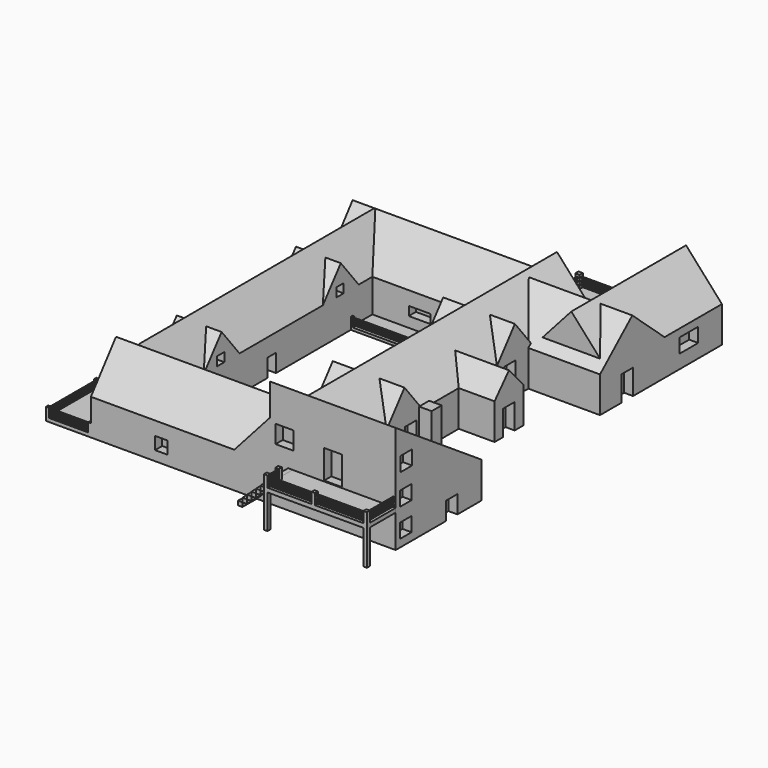
from build123d import *

# Parameters (mm, degrees)
F0_W       = 101.6
F0_H       = 50.8
F1_DEPTH   = 508
F2_W       = 152.4
F2_H       = 50.8
F3_DEPTH   = 127
F4_DEPTH   = 127
F5_DEPTH   = 50.8
F6_W       = 50.8
F6_H       = 50.8
F7_DEPTH   = 50.8
F8_DEPTH   = 25.4
F9_W       = 114.3
F9_H       = 50.8
F10_DEPTH  = 101.6
F11_DEPTH  = 50.8
F12_W      = 101.6
F12_H      = 50.8
F13_DEPTH  = 101.6
F14_DEPTH  = 101.6
F15_W      = 88.9
F15_H      = 50.8
F16_DEPTH  = 203.2
F17_DEPTH  = 50.8
F18_DEPTH  = 50.8
F19_W      = 63.5
F19_H      = 50.8
F20_DEPTH  = 355.6
F21_DEPTH  = 17.78
F22_DEPTH  = 43.18
F24_DEPTH  = 101.6
F26_DEPTH  = 63.5
F27_W      = 101.6
F27_H      = 7.62
F28_DEPTH  = 101.6
F29_W      = 6.096
F29_H      = 5.588
F30_DEPTH  = 17.78
F31_W      = 1.524
F31_H      = 1.397
F32_DEPTH  = 63.5
F33_W      = 1.524
F33_H      = 1.397
F34_DEPTH  = 127
F35_W      = 5.08
F35_H      = 3.81
F36_DEPTH  = 30.48
F37_W      = 6.35
F37_H      = 5.842
F38_DEPTH  = 25.4
F37_W_2    = 146.05
F39_DEPTH  = 50.8
F40_W      = 5.08
F40_H      = 5.08
F41_DEPTH  = 15.24
F42_W      = 1.778
F42_H      = 1.778
F43_DEPTH  = 139.7
F44_W      = 1.778
F44_H      = 1.778
F45_DEPTH  = 50.8
F46_W      = 1.778
F46_H      = 1.778
F47_DEPTH  = 17.78
F48_W      = 330.2
F48_H      = 3.81
F49_DEPTH  = 38.1
F50_W      = 101.6
F50_H      = 3.81
F51_DEPTH  = 38.1
F52_W      = 101.6
F52_H      = 3.81
F53_DEPTH  = 38.1
F54_W      = 15.24
F54_H      = 2.54
F55_DEPTH  = 2.54
F56_W      = 3.048
F56_H      = 3.048
F57_DEPTH  = 12.7
F58_W      = 1.27
F58_H      = 1.27
F62_DEPTH  = 101.6
F59_W      = 1.27
F59_H      = 1.27
F63_DEPTH  = 109.22
F60_W      = 1.27
F60_H      = 1.27
F64_DEPTH  = 127
F61_W      = 1.27
F61_H      = 1.27
F65_DEPTH  = 101.6
F66_W      = 17.78
F66_H      = 17.78
F67_DEPTH  = 114.3
F70_DEPTH  = 63.5
F69_W      = 20.32
F69_H      = 38.1
F69_W_2    = 17.78
F69_H_2    = 17.78
F69_W_3    = 17.272
F69_H_3    = 35.56
F78_DEPTH  = 12.7
F71_W      = 20.32
F71_H      = 35.56
F71_W_2    = 12.7
F71_H_2    = 12.7
F79_DEPTH  = 12.7
F72_W      = 40.64
F72_H      = 15.24
F80_DEPTH  = 12.7
F73_W      = 33.02
F73_H      = 20.32
F81_DEPTH  = 12.7
F74_W      = 20.32
F74_H      = 35.56
F74_W_2    = 33.02
F74_H_2    = 20.32
F82_DEPTH  = 12.7
F75_W      = 20.32
F75_H      = 20.32
F83_DEPTH  = 12.7
F76_W      = 20.32
F76_H      = 35.56
F84_DEPTH  = 12.7
F77_W      = 20.32
F77_H      = 20.32
F77_H_2    = 25.4
F85_DEPTH  = 12.7
F68_W      = 25.4
F68_H      = 25.4
F68_H_2    = 40.64
F86_DEPTH  = 12.7
F87_W      = 20.32
F87_H      = 25.4
F87_W_2    = 15.24
F87_H_2    = 15.24
F91_DEPTH  = 12.7
F88_W      = 30.48
F88_H      = 12.7
F92_DEPTH  = 12.7
F89_W      = 12.7
F89_H      = 12.7
F89_W_2    = 15.24
F89_H_2    = 25.4
F93_DEPTH  = 12.7
F90_W      = 30.48
F90_H      = 12.7
F94_DEPTH  = 12.7
F95_W      = 3.81
F95_H      = 3.81
F96_DEPTH  = 12.7
F97_W      = 1.524
F97_H      = 1.524
F100_DEPTH = 58.42
F99_W      = 1.524
F99_H      = 1.524
F101_DEPTH = 81.28
F98_W      = 1.524
F98_H      = 1.524
F102_DEPTH = 58.42
F103_W     = 3.81
F103_H     = 3.81
F104_DEPTH = 12.7
F105_W     = 1.524
F105_H     = 1.524
F108_DEPTH = 58.42
F106_W     = 1.524
F106_H     = 1.524
F109_DEPTH = 83.82
F107_W     = 1.524
F107_H     = 1.524
F110_DEPTH = 58.42
F111_W     = 5.08
F111_H     = 5.08
F112_DEPTH = 48.26
F68_W_2    = 17.78
F68_H_3    = 17.78
F113_DEPTH = 12.7


# Not quite as in the source:
# - a feature names something its author has since deleted; it is built from what else it names


with BuildPart() as f1:
    # F0 (on Front) → F1 (new body)
    with BuildSketch(Plane.XZ):
        Polygon((0, 56.7961266285), (-50.8, 0), (50.8, 0), align=None)
        with Locations((0, -25.4)):
            Rectangle(F0_W, F0_H)
    extrude(amount=F1_DEPTH)

    # F2 (on face) → F3 (join)
    with BuildSketch(Plane.YZ.offset(50.8)):
        with Locations((-431.8, -25.4)):
            Rectangle(F2_W, F2_H)
    extrude(amount=F3_DEPTH)

    # F2 (on face) → F4 (join)
    with BuildSketch(Plane.YZ.offset(50.8)):
        Polygon((-508, 0), (-355.6, 0), (-508, 101.6), align=None)
    extrude(amount=F4_DEPTH)

    # F5 (add): a face of the model
    f5_faces = [f1.faces().sort_by_distance(p)[0] for p in [
        (50.8, -457.2, 33.8666666667),
    ]]
    extrude(f5_faces, amount=F5_DEPTH)

    # F6 (on face) → F7 (join)
    with BuildSketch(Plane.YZ.offset(50.8)):
        with Locations((-212.1169992447, -25.4)):
            Rectangle(F6_W, F6_H)
        Polygon((-212.1169992447, 28.3980633142), (-237.5169992447, 0), (-186.7169992447, 0), align=None)
    extrude(amount=F7_DEPTH)

    # F8 (add): a face of the model
    f8_faces = [f1.faces().sort_by_distance(p)[0] for p in [
        (50.8, -212.1169992447, 9.4660211047),
    ]]
    extrude(f8_faces, amount=F8_DEPTH)

    # F9 (on face) → F10 (join)
    with BuildSketch(Plane.YZ.offset(50.8)):
        Polygon((-57.15, 50.4015624758), (-114.3, 0), (0, 0), align=None)
        with Locations((-57.15, -25.4)):
            Rectangle(F9_W, F9_H)
    extrude(amount=F10_DEPTH)

    # F11 (add): a face of the model
    f11_faces = [f1.faces().sort_by_distance(p)[0] for p in [
        (50.8, -57.15, 16.8005208253),
    ]]
    extrude(f11_faces, amount=F11_DEPTH)

    # F12 (on face) → F13 (join)
    with BuildSketch(Plane(origin=(0, 0, 0), x_dir=(-1, 0, 0), z_dir=(0, 1, 0))):
        with Locations((-101.6, -25.4)):
            Rectangle(F12_W, F12_H)
        Polygon((-152.4, 0), (-50.8, 0), (-101.6, 56.7961266285), align=None)
    extrude(amount=F13_DEPTH)

    # F14 (add): a face of the model
    f14_faces = [f1.faces().sort_by_distance(p)[0] for p in [
        (101.6, 0, 18.9320422095),
    ]]
    extrude(f14_faces, amount=F14_DEPTH)

    # F15 (on face) → F16 (join)
    with BuildSketch(Plane(origin=(-50.8, 0, 0), x_dir=(0, -1, 0), z_dir=(-1, 0, 0))):
        with Locations((44.45, -25.4)):
            Rectangle(F15_W, F15_H)
        Polygon((44.45, 56.8137306995), (0, 0), (88.9, 0), align=None)
        with Locations((463.55, -25.4)):
            Rectangle(F15_W, F15_H)
        Polygon((463.55, 56.8137306995), (419.1, 0), (508, 0), align=None)
    extrude(amount=F16_DEPTH)

    # F17 (add): a face of the model
    f17_faces = [f1.faces().sort_by_distance(p)[0] for p in [
        (-50.8, -44.45, 18.9379102332),
    ]]
    extrude(f17_faces, amount=F17_DEPTH)

    # F18 (add): a face of the model
    f18_faces = [f1.faces().sort_by_distance(p)[0] for p in [
        (-50.8, -463.55, 18.9379102332),
    ]]
    extrude(f18_faces, amount=F18_DEPTH)

    # F19 (on face) → F20 (join)
    with BuildSketch(Plane.XZ.offset(88.9)):
        with Locations((-222.25, -25.4)):
            Rectangle(F19_W, F19_H)
        Polygon((-254, 0), (-190.5, 0), (-222.25, 57.6171441153), align=None)
    extrude(amount=F20_DEPTH)

    # F21 (add): a face of the model
    f21_faces = [f1.faces().sort_by_distance(p)[0] for p in [
        (-222.25, -444.5, 40.8490406859),
    ]]
    extrude(f21_faces, amount=F21_DEPTH)

    # F22 (add): a face of the model
    f22_faces = [f1.faces().sort_by_distance(p)[0] for p in [
        (-222.25, -88.9, 19.2057147051),
    ]]
    extrude(f22_faces, amount=F22_DEPTH)

    # F23 (on face) → F24 (join)
    with BuildSketch(Plane(origin=(-50.8, 0, 0), x_dir=(0, -1, 0), z_dir=(-1, 0, 0))):
        Polygon((138.0952139497, 39.6557372898), (106.3452139497, 0), (169.8452139497, 0), align=None)
        Polygon((333.6137141702, 39.6557372898), (301.8637141702, 0), (365.3637141702, 0), align=None)
    extrude(amount=-F24_DEPTH)

    # F25 (on face) → F26 (join)
    with BuildSketch(Plane(origin=(-254, 0, 0), x_dir=(0, -1, 0), z_dir=(-1, 0, 0))):
        Polygon((144.8305835128, 39.6557372898), (113.0805835128, 0), (176.5805835128, 0), align=None)
        Polygon((355.9101884365, 39.6557372898), (324.1601884365, 0), (387.6601884365, 0), align=None)
    extrude(amount=-F26_DEPTH)

    # F27 (on face) → F28 (join)
    with BuildSketch(Plane(origin=(50.8, 0, 0), x_dir=(0, -1, 0), z_dir=(-1, 0, 0))):
        with Locations((-50.8, -46.99)):
            Rectangle(F27_W, F27_H)
    extrude(amount=F28_DEPTH)

    # F29 (on face) → F30 (join)
    with BuildSketch(Plane.XY.offset(-43.18)):
        with Locations((-47.752, 33.3146086487)):
            Rectangle(F29_W, F29_H)
        with Locations((-47.752, 98.806)):
            Rectangle(F29_W, F29_H)
        with Locations((6.6813429161, 98.806)):
            Rectangle(F29_W, F29_H)
    extrude(amount=F30_DEPTH)

    # F31 (on face) → F32 (join)
    with BuildSketch(Plane(origin=(0, 36.1086086487, 0), x_dir=(-1, 0, 0), z_dir=(0, 1, 0))):
        with Locations((47.498, -38.7985)):
            Rectangle(F31_W, F31_H)
        with Locations((47.498, -34.0995)):
            Rectangle(F31_W, F31_H)
        with Locations((47.498, -29.4005)):
            Rectangle(F31_W, F31_H)
    extrude(amount=F32_DEPTH)

    # F33 (on face) → F34 (join)
    with BuildSketch(Plane.YZ.offset(-44.704)):
        with Locations((98.806, -29.4005)):
            Rectangle(F33_W, F33_H)
        with Locations((98.806, -34.0995)):
            Rectangle(F33_W, F33_H)
        with Locations((98.806, -38.7985)):
            Rectangle(F33_W, F33_H)
    extrude(amount=F34_DEPTH)

    # F35 (on face) → F36 (join)
    with BuildSketch(Plane(origin=(0, 0, 0), x_dir=(-1, 0, 0), z_dir=(0, 1, 0))):
        with Locations((53.34, -48.895)):
            Rectangle(F35_W, F35_H)
    extrude(amount=F36_DEPTH)

    # F48 (on face) → F49 (join)
    with BuildSketch(Plane(origin=(-50.8, 0, 0), x_dir=(0, -1, 0), z_dir=(-1, 0, 0))):
        with Locations((254, -48.895)):
            Rectangle(F48_W, F48_H)
    extrude(amount=F49_DEPTH)

    # F50 (on face) → F51 (join)
    with BuildSketch(Plane.XZ.offset(88.9)):
        with Locations((-139.7, -48.895)):
            Rectangle(F50_W, F50_H)
    extrude(amount=F51_DEPTH)

    # F52 (on face) → F53 (join)
    with BuildSketch(Plane(origin=(0, -419.1, 0), x_dir=(-1, 0, 0), z_dir=(0, 1, 0))):
        with Locations((139.7, -48.895)):
            Rectangle(F52_W, F52_H)
    extrude(amount=F53_DEPTH)

    # F54 (on face) → F55 (join)
    with BuildSketch(Plane(origin=(-88.9, 0, 0), x_dir=(0, -1, 0), z_dir=(-1, 0, 0))):
        with Locations((246.4711151075, -49.53)):
            Rectangle(F54_W, F54_H)
    extrude(amount=F55_DEPTH)

    # F56 (on face) → F57 (join)
    with BuildSketch(Plane.XY.offset(-46.99)):
        with Locations((-188.976, -125.476)):
            Rectangle(F56_W, F56_H)
        with Locations((-87.376, -125.476)):
            Rectangle(F56_W, F56_H)
        with Locations((-87.376, -237.3516275177)):
            Rectangle(F56_W, F56_H)
        with Locations((-87.376, -255.524)):
            Rectangle(F56_W, F56_H)
        with Locations((-87.376, -382.524)):
            Rectangle(F56_W, F56_H)
        with Locations((-188.976, -382.524)):
            Rectangle(F56_W, F56_H)
    extrude(amount=F57_DEPTH)

    # F58 (on face) → F62 (join)
    with BuildSketch(Plane.YZ.offset(-187.452)):
        with Locations((-125.349, -36.195)):
            Rectangle(F58_W, F58_H)
        with Locations((-125.349, -40.005)):
            Rectangle(F58_W, F58_H)
        with Locations((-125.349, -43.815)):
            Rectangle(F58_W, F58_H)
    extrude(amount=F62_DEPTH)

    # F59 (on face) → F63 (join)
    with BuildSketch(Plane.XZ.offset(127)):
        with Locations((-87.249, -36.195)):
            Rectangle(F59_W, F59_H)
        with Locations((-87.249, -40.005)):
            Rectangle(F59_W, F59_H)
        with Locations((-87.249, -43.815)):
            Rectangle(F59_W, F59_H)
    extrude(amount=F63_DEPTH)

    # F60 (on face) → F64 (join)
    with BuildSketch(Plane.XZ.offset(257.048)):
        with Locations((-87.249, -36.195)):
            Rectangle(F60_W, F60_H)
        with Locations((-87.249, -40.005)):
            Rectangle(F60_W, F60_H)
        with Locations((-87.249, -43.815)):
            Rectangle(F60_W, F60_H)
    extrude(amount=F64_DEPTH)

    # F61 (on face) → F65 (join)
    with BuildSketch(Plane(origin=(-88.9, 0, 0), x_dir=(0, -1, 0), z_dir=(-1, 0, 0))):
        with Locations((382.651, -36.195)):
            Rectangle(F61_W, F61_H)
        with Locations((382.6914110303, -40.0046785129)):
            Rectangle(F61_W, F61_H)
        with Locations((382.651, -43.8146785129)):
            Rectangle(F61_W, F61_H)
    extrude(amount=F65_DEPTH)

    # F66 (on face) → F67 (join)
    with BuildSketch(Plane(origin=(0, 0, -50.8), x_dir=(1, 0, 0), z_dir=(0, 0, -1))):
        with Locations((129.2515342133, 385.8176767826)):
            Rectangle(F66_W, F66_H)
    extrude(amount=-F67_DEPTH)

    # F69 (on face) → F70 (join)
    with BuildSketch(Plane(origin=(-254, 0, 0), x_dir=(0, -1, 0), z_dir=(-1, 0, 0))):
        Polygon((0, -50.8), (88.9, -50.8), (88.9, -45.72), (49.4282281619, -45.72), (29.1082281619, -45.72), (0, -45.72), align=None)
        Polygon((419.1, -45.72), (419.1, -50.8), (508, -50.8), (508, -45.72), (471.0614698601, -45.72), (450.7414698601, -45.72), align=None)
    extrude(amount=F70_DEPTH)

    # F69 (on face) → F78 (cut)
    with BuildSketch(Plane(origin=(-254, 0, 0), x_dir=(0, -1, 0), z_dir=(-1, 0, 0))):
        with Locations((39.2682281619, -26.67)):
            Rectangle(F69_W, F69_H)
        with Locations((144.3404865994, 8.89)):
            Rectangle(F69_W_2, F69_H_2)
        with Locations((230.9999394188, -33.02)):
            Rectangle(F69_W_3, F69_H_3)
        with Locations((252.8439394188, -33.02)):
            Rectangle(F69_W, F69_H_3)
        with Locations((355.4200915231, 8.89)):
            Rectangle(F69_W_2, F69_H_2)
        with Locations((460.9014698601, -26.67)):
            Rectangle(F69_W, F69_H)
    extrude(amount=-F78_DEPTH, mode=Mode.SUBTRACT)

    # F71 (on face) → F79 (cut)
    with BuildSketch(Plane(origin=(0, 0, 0), x_dir=(-1, 0, 0), z_dir=(0, 1, 0))):
        with Locations((-10.16, -25.4)):
            Rectangle(F71_W, F71_H)
        with Locations((96.6436273593, -13.97)):
            Rectangle(F71_W_2, F71_H_2)
        with Locations((192.706280126, -13.97)):
            Rectangle(F71_W_2, F71_H_2)
    extrude(amount=-F79_DEPTH, mode=Mode.SUBTRACT)

    # F72 (on face) → F80 (cut)
    with BuildSketch(Plane(origin=(50.8, 0, 0), x_dir=(0, -1, 0), z_dir=(-1, 0, 0))):
        with Locations((-47.1025463194, -21.7962798297)):
            Rectangle(F72_W, F72_H)
    extrude(amount=-F80_DEPTH, mode=Mode.SUBTRACT)

    # F73 (on face) → F81 (cut)
    with BuildSketch(Plane(origin=(0, 101.6, 0), x_dir=(-1, 0, 0), z_dir=(0, 1, 0))):
        with Locations((-103.4534499049, -6.6979110748)):
            Rectangle(F73_W, F73_H)
    extrude(amount=-F81_DEPTH, mode=Mode.SUBTRACT)

    # F74 (on face) → F82 (cut)
    with BuildSketch(Plane.YZ.offset(152.4)):
        with Locations((-65.913564589, -33.02)):
            Rectangle(F74_W, F74_H)
        with Locations((43.0610267541, -21.277274017)):
            Rectangle(F74_W_2, F74_H_2)
    extrude(amount=-F82_DEPTH, mode=Mode.SUBTRACT)

    # F75 (on face) → F83 (cut)
    with BuildSketch(Plane.YZ.offset(50.8)):
        with Locations((-147.4105939269, -16.3445944426)):
            Rectangle(F75_W, F75_H)
        with Locations((-322.6297489071, -19.8411597574)):
            Rectangle(F75_W, F75_H)
    extrude(amount=-F83_DEPTH, mode=Mode.SUBTRACT)

    # F76 (on face) → F84 (cut)
    with BuildSketch(Plane.YZ.offset(101.6)):
        with Locations((-212.1169992447, -33.02)):
            Rectangle(F76_W, F76_H)
    extrude(amount=-F84_DEPTH, mode=Mode.SUBTRACT)

    # F77 (on face) → F85 (cut)
    with BuildSketch(Plane.YZ.offset(177.8)):
        with Locations((-489.0044620895, 52.9891969001)):
            Rectangle(F77_W, F77_H)
        with Locations((-489.8959687614, 10.16)):
            Rectangle(F77_W, F77_H)
        with Locations((-490.0082043076, -29.826025542)):
            Rectangle(F77_W, F77_H)
        with Locations((-408.7290457153, -38.1)):
            Rectangle(F77_W, F77_H_2)
    extrude(amount=-F85_DEPTH, mode=Mode.SUBTRACT)

    # F68 (on face) → F86 (cut)
    with BuildSketch(Plane.XZ.offset(508)):
        with Locations((20.4100181952, 38.7479077697)):
            Rectangle(F68_W, F68_H)
        with Locations((89.1670092579, 23.3091599075)):
            Rectangle(F68_W, F68_H_2)
    extrude(amount=-F86_DEPTH, mode=Mode.SUBTRACT)

    # F87 (on face) → F91 (cut)
    with BuildSketch(Plane(origin=(-50.8, 0, 0), x_dir=(0, -1, 0), z_dir=(-1, 0, 0))):
        with Locations((138.3743443823, -34.29)):
            Rectangle(F87_W, F87_H)
        with Locations((194.9318728399, -18.4517626661)):
            Rectangle(F87_W_2, F87_H_2)
        with Locations((276.5751115036, -18.4517626661)):
            Rectangle(F87_W_2, F87_H_2)
        with Locations((333.6193570232, -34.29)):
            Rectangle(F87_W, F87_H)
    extrude(amount=-F91_DEPTH, mode=Mode.SUBTRACT)

    # F88 (on face) → F92 (cut)
    with BuildSketch(Plane.XZ.offset(88.9)):
        with Locations((-123.6675304985, -25.8926844908)):
            Rectangle(F88_W, F88_H)
    extrude(amount=-F92_DEPTH, mode=Mode.SUBTRACT)

    # F89 (on face) → F93 (cut)
    with BuildSketch(Plane.YZ.offset(-190.5)):
        with Locations((-357.4289785862, 6.35)):
            Rectangle(F89_W, F89_H)
        with Locations((-267.2483094978, -38.1)):
            Rectangle(F89_W_2, F89_H_2)
        with Locations((-146.1940599442, 6.35)):
            Rectangle(F89_W, F89_H)
    extrude(amount=-F93_DEPTH, mode=Mode.SUBTRACT)

    # F90 (on face) → F94 (cut)
    with BuildSketch(Plane(origin=(0, -419.1, 0), x_dir=(-1, 0, 0), z_dir=(0, 1, 0))):
        with Locations((125.8972622454, -24.3402836923)):
            Rectangle(F90_W, F90_H)
    extrude(amount=-F94_DEPTH, mode=Mode.SUBTRACT)

    # F95 (on face) → F96 (join)
    with BuildSketch(Plane.XY.offset(-45.72)):
        with Locations((-315.595, -1.905)):
            Rectangle(F95_W, F95_H)
        with Locations((-255.905, -86.995)):
            Rectangle(F95_W, F95_H)
        with Locations((-315.595, -86.995)):
            Rectangle(F95_W, F95_H)
        with Locations((-255.905, -1.905)):
            Rectangle(F95_W, F95_H)
    extrude(amount=F96_DEPTH)

    # F97 (on face) → F100 (join)
    with BuildSketch(Plane(origin=(-257.81, 0, 0), x_dir=(0, -1, 0), z_dir=(-1, 0, 0))):
        with Locations((1.778, -35.56)):
            Rectangle(F97_W, F97_H)
        with Locations((1.778, -39.624)):
            Rectangle(F97_W, F97_H)
        with Locations((1.778, -43.688)):
            Rectangle(F97_W, F97_H)
    extrude(amount=F100_DEPTH)

    # F99 (on face) → F101 (join)
    with BuildSketch(Plane.XZ.offset(3.81)):
        with Locations((-315.722, -35.56)):
            Rectangle(F99_W, F99_H)
        with Locations((-315.722, -39.624)):
            Rectangle(F99_W, F99_H)
        with Locations((-315.722, -43.688)):
            Rectangle(F99_W, F99_H)
    extrude(amount=F101_DEPTH)

    # F98 (on face) → F102 (join)
    with BuildSketch(Plane(origin=(-257.81, 0, 0), x_dir=(0, -1, 0), z_dir=(-1, 0, 0))):
        with Locations((86.868, -35.56)):
            Rectangle(F98_W, F98_H)
        with Locations((86.868, -39.624)):
            Rectangle(F98_W, F98_H)
        with Locations((86.868, -43.688)):
            Rectangle(F98_W, F98_H)
    extrude(amount=F102_DEPTH)

    # F103 (on face) → F104 (join)
    with BuildSketch(Plane.XY.offset(-45.72)):
        with Locations((-315.595, -421.005)):
            Rectangle(F103_W, F103_H)
        with Locations((-255.905, -421.005)):
            Rectangle(F103_W, F103_H)
        with Locations((-315.595, -506.095)):
            Rectangle(F103_W, F103_H)
        with Locations((-255.905, -506.095)):
            Rectangle(F103_W, F103_H)
    extrude(amount=F104_DEPTH)

    # F105 (on face) → F108 (join)
    with BuildSketch(Plane(origin=(-257.81, 0, 0), x_dir=(0, -1, 0), z_dir=(-1, 0, 0))):
        with Locations((420.878, -35.56)):
            Rectangle(F105_W, F105_H)
        with Locations((420.878, -39.624)):
            Rectangle(F105_W, F105_H)
        with Locations((420.878, -43.688)):
            Rectangle(F105_W, F105_H)
    extrude(amount=F108_DEPTH)

    # F106 (on face) → F109 (join)
    with BuildSketch(Plane.XZ.offset(422.91)):
        with Locations((-315.722, -35.56)):
            Rectangle(F106_W, F106_H)
        with Locations((-315.722, -39.624)):
            Rectangle(F106_W, F106_H)
        with Locations((-315.722, -43.688)):
            Rectangle(F106_W, F106_H)
    extrude(amount=F109_DEPTH)

    # F107 (on face) → F110 (join)
    with BuildSketch(Plane(origin=(-257.81, 0, 0), x_dir=(0, -1, 0), z_dir=(-1, 0, 0))):
        with Locations((505.968, -35.56)):
            Rectangle(F107_W, F107_H)
        with Locations((505.968, -39.624)):
            Rectangle(F107_W, F107_H)
        with Locations((505.968, -43.688)):
            Rectangle(F107_W, F107_H)
    extrude(amount=F110_DEPTH)

    # F68 (on face) → F113 (cut)
    with BuildSketch(Plane.XZ.offset(508)):
        with Locations((-154.2257547235, -28.1168065822)):
            Rectangle(F68_W_2, F68_H_3)
    extrude(amount=-F113_DEPTH, mode=Mode.SUBTRACT)


with BuildPart() as f38:
    # F37 (on face) → F38 (new body)
    with BuildSketch(Plane.XZ.offset(508)):
        with Locations((-15.875, -42.037)):
            Rectangle(F37_W, F37_H)
    extrude(amount=F38_DEPTH)


with BuildPart() as f38b:
    # F37 (on face) → F38, piece 2 (new body)
    with BuildSketch(Plane.XZ.offset(508)):
        with Locations((-22.225, -47.879)):
            Rectangle(F37_W, F37_H)
    extrude(amount=F38_DEPTH)


with BuildPart() as f38c:
    # F37 (on face) → F38, piece 3 (new body)
    with BuildSketch(Plane.XZ.offset(508)):
        with Locations((-9.525, -36.195)):
            Rectangle(F37_W, F37_H)
    extrude(amount=F38_DEPTH)


with BuildPart() as f38d:
    # F37 (on face) → F38, piece 4 (new body)
    with BuildSketch(Plane.XZ.offset(508)):
        with Locations((-3.175, -30.353)):
            Rectangle(F37_W, F37_H)
    extrude(amount=F38_DEPTH)


with BuildPart() as f38e:
    # F37 (on face) → F38, piece 5 (new body)
    with BuildSketch(Plane.XZ.offset(508)):
        with Locations((3.175, -24.511)):
            Rectangle(F37_W, F37_H)
    extrude(amount=F38_DEPTH)


with BuildPart() as f38f:
    # F37 (on face) → F38, piece 6 (new body)
    with BuildSketch(Plane.XZ.offset(508)):
        with Locations((9.525, -18.669)):
            Rectangle(F37_W, F37_H)
    extrude(amount=F38_DEPTH)


with BuildPart() as f38g:
    # F37 (on face) → F38, piece 7 (new body)
    with BuildSketch(Plane.XZ.offset(508)):
        with Locations((15.875, -12.827)):
            Rectangle(F37_W, F37_H)
    extrude(amount=F38_DEPTH)


with BuildPart() as f38h:
    # F37 (on face) → F38, piece 8 (new body)
    with BuildSketch(Plane.XZ.offset(508)):
        with Locations((22.225, -6.985)):
            Rectangle(F37_W, F37_H)
    extrude(amount=F38_DEPTH)


with BuildPart() as f38i:
    # F37 (on face) → F38, piece 9 (new body)
    with BuildSketch(Plane.XZ.offset(508)):
        with Locations((28.575, -1.143)):
            Rectangle(F37_W, F37_H)
    extrude(amount=F38_DEPTH)


with BuildPart() as f39:
    # F37 (on face) → F39 (new body)
    with BuildSketch(Plane.XZ.offset(508)):
        with Locations((104.775, -1.143)):
            Rectangle(F37_W_2, F37_H)
    extrude(amount=F39_DEPTH)

    # F40 (on face) → F41 (join)
    with BuildSketch(Plane.XY.offset(1.778)):
        with Locations((34.29, -535.94)):
            Rectangle(F40_W, F40_H)
        with Locations((34.29, -556.26)):
            Rectangle(F40_W, F40_H)
        with Locations((101.7828585887, -556.26)):
            Rectangle(F40_W, F40_H)
        with Locations((175.26, -556.26)):
            Rectangle(F40_W, F40_H)
    extrude(amount=F41_DEPTH)

    # F42 (on face) → F43 (join)
    with BuildSketch(Plane.YZ.offset(36.83)):
        with Locations((-556.133, 13.589)):
            Rectangle(F42_W, F42_H)
        with Locations((-556.133, 8.8574167275)):
            Rectangle(F42_W, F42_H)
        with Locations((-556.133, 4.4352533091)):
            Rectangle(F42_W, F42_H)
    extrude(amount=F43_DEPTH)

    # F46 (on face) → F47 (join)
    with BuildSketch(Plane.XZ.offset(538.48)):
        with Locations((34.417, 13.589)):
            Rectangle(F46_W, F46_H)
        with Locations((34.417, 9.271)):
            Rectangle(F46_W, F46_H)
        with Locations((34.417, 5.207)):
            Rectangle(F46_W, F46_H)
    extrude(amount=F47_DEPTH)

    # F111 (on face) → F112 (join)
    with BuildSketch(Plane(origin=(0, 0, -4.064), x_dir=(1, 0, 0), z_dir=(0, 0, -1))):
        with Locations((175.26, 556.26)):
            Rectangle(F111_W, F111_H)
        with Locations((34.29, 556.26)):
            Rectangle(F111_W, F111_H)
    extrude(amount=F112_DEPTH)


with BuildPart() as f45:
    # F44 (on face) → F45 (new body)
    with BuildSketch(Plane(origin=(0, -553.72, 0), x_dir=(-1, 0, 0), z_dir=(0, 1, 0))):
        with Locations((-175.133, 13.9625315124)):
            Rectangle(F44_W, F44_H)
    extrude(amount=F45_DEPTH)


with BuildPart() as f45b:
    # F44 (on face) → F45, piece 2 (new body)
    with BuildSketch(Plane(origin=(0, -553.72, 0), x_dir=(-1, 0, 0), z_dir=(0, 1, 0))):
        with Locations((-175.133, 9.7249951795)):
            Rectangle(F44_W, F44_H)
    extrude(amount=F45_DEPTH)


with BuildPart() as f45c:
    # F44 (on face) → F45, piece 3 (new body)
    with BuildSketch(Plane(origin=(0, -553.72, 0), x_dir=(-1, 0, 0), z_dir=(0, 1, 0))):
        with Locations((-175.133, 4.6899936399)):
            Rectangle(F44_W, F44_H)
    extrude(amount=F45_DEPTH)


solid = Compound([f1.part, f38.part, f38b.part, f38c.part, f38d.part, f38e.part, f38f.part, f38g.part, f38h.part, f38i.part, f39.part, f45.part, f45b.part, f45c.part])
